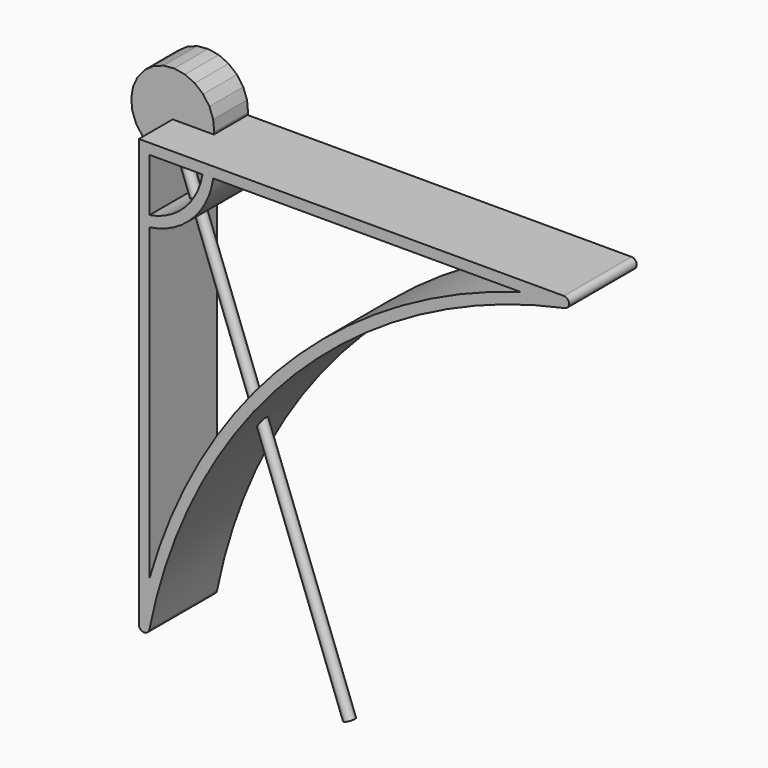
from build123d import *

# Parameters (mm, degrees)
F1_DEPTH = 50.8
F3_DEPTH = 25.4
F6_DEPTH = 279.4


with BuildPart() as f1:
    # F0 (on Front) → F1 (new body)
    with BuildSketch(Plane.XZ):
        with BuildLine():
            Line((0, 320.5072749112), (0, 63.8402879052))
            ThreePointArc((0, 63.8402879052), (2.8607431223, 60.6808785276), (6.2877906235, 63.214860424))
            ThreePointArc((6.2877906235, 63.214860424), (93.2857648732, 226.2096554871), (255.734288563, 314.2234492481))
            ThreePointArc((255.734288563, 314.2234492481), (258.247854386, 317.6563918034), (255.0894412971, 320.5072749112))
            Line((255.0894412971, 320.5072749112), (0, 320.5072749112))
        make_face()
        with BuildLine():
            Line((6.35, 275.8740514516), (6.35, 282.2986734306))
            Line((6.35, 282.2986734306), (6.35, 314.1572749112))
            Line((6.35, 314.1572749112), (38.2086014806, 314.1572749112))
            Line((38.2086014806, 314.1572749112), (44.6332234596, 314.1572749112))
            Line((44.6332234596, 314.1572749112), (229.2298219421, 314.1572749112))
            ThreePointArc((229.2298219421, 314.1572749112), (88.988701653, 230.893914438), (6.35, 90.2838009813))
            Line((6.35, 90.2838009813), (6.35, 275.8740514516))
        make_face(mode=Mode.SUBTRACT)
        with BuildLine():
            ThreePointArc((38.2086014806, 314.1572749112), (27.3881336266, 293.1191412846), (6.35, 282.2986734306))
            Line((6.35, 282.2986734306), (6.35, 275.8740514516))
            ThreePointArc((6.35, 275.8740514516), (31.8782616872, 288.629013224), (44.6332234596, 314.1572749112))
            Line((44.6332234596, 314.1572749112), (38.2086014806, 314.1572749112))
        make_face()
    extrude(amount=F1_DEPTH)

    # F4 (on face) → F6 (join)
    with BuildSketch(Plane(origin=(-96.9764298817, 0, 260.3424117621), x_dir=(0.9370984586, 0, 0.3490651498), z_dir=(0.3490651498, 0, -0.9370984586))):
        with BuildLine():
            Line((109.5114211305, 25.4), (115.8614211305, 25.4))
            ThreePointArc((115.8614211305, 25.4), (112.6864211305, 28.575), (109.5114211305, 25.4))
        make_face()
        with BuildLine():
            ThreePointArc((109.5114211305, 25.4), (112.6864211305, 22.225), (115.8614211305, 25.4))
            Line((115.8614211305, 25.4), (109.5114211305, 25.4))
        make_face()
    extrude(amount=F6_DEPTH)


with BuildPart() as f3:
    # F2 (on Front) → F3 (new body)
    with BuildSketch(Plane.XZ):
        Polygon((24.2812376232, 328.3980579991), (22.0110636442, 334.49255508), (18.2408720527, 339.7918229472), (13.2275951754, 343.934725253), (7.3128795465, 346.6389300518), (0.8998032616, 347.7201502554), (-5.5745931286, 347.1047024937), (-11.6690902095, 344.8345285146), (-16.9683580768, 341.0643369232), (-21.1112603826, 336.0510600458), (-23.8154651814, 330.1363444169), (-24.8966853849, 323.723268132), (-24.2812376232, 317.2488717418), (-22.0110636442, 311.1543746609), (-18.2408720527, 305.8551067937), (-13.2275951754, 301.7122044879), (-7.3128795465, 299.0079996891), (-0.8998032616, 297.9267794855), (5.5745931286, 298.5422272472), (11.6690902095, 300.8124012263), (16.9683580768, 304.5825928177), (21.1112603826, 309.5958696951), (23.8154651814, 315.510585324), (24.8966853849, 321.9236616089), align=None)
    extrude(amount=F3_DEPTH)


solid = Compound([f1.part, f3.part])
